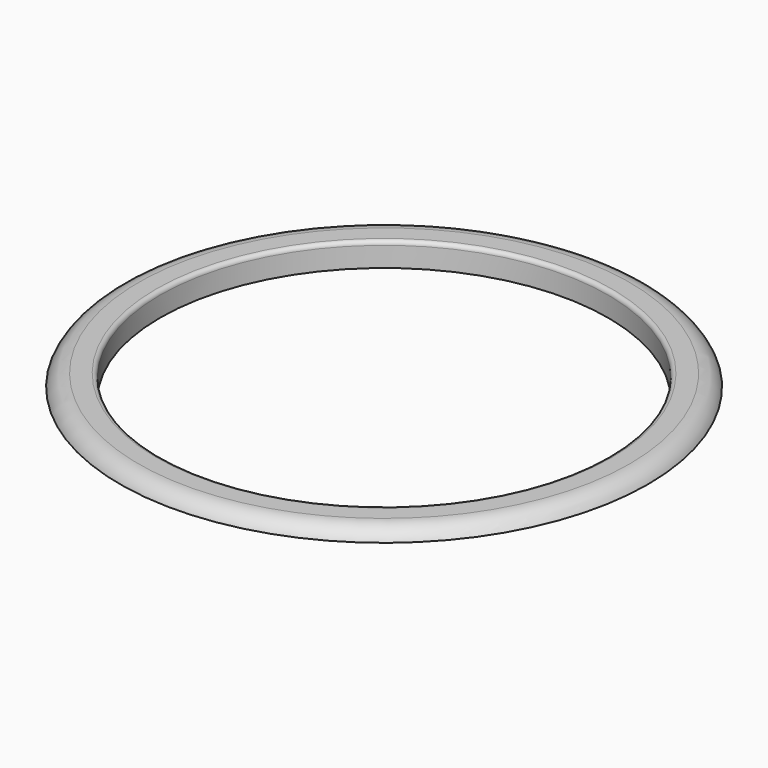
from build123d import *

# Parameters (mm, degrees)
F0_R     = 58
F0_R_2   = 56
F1_DEPTH = 3
F2_R     = 66
F2_R_2   = 58
F2_R_3   = 56
F3_DEPTH = 3
F5_R     = 1


# Not quite as in the source:
# - a fillet or chamfer that OpenCascade refuses, or shapes differently, is made with other operations: its cross-section is extruded or revolved along the edge and cut away or added


with BuildPart() as f1:
    # F0 (on Top) → F1 (new body)
    with BuildSketch(Plane.XY):
        Circle(F0_R)
        Circle(F0_R_2, mode=Mode.SUBTRACT)
    extrude(amount=F1_DEPTH)

    # F2 (on face) → F3 (join)
    with BuildSketch(Plane.XY.offset(3)):
        Circle(F2_R)
        Circle(F2_R_2, mode=Mode.SUBTRACT)
        Circle(F2_R_2)
        Circle(F2_R_3, mode=Mode.SUBTRACT)
    extrude(amount=F3_DEPTH)

    # F4: fillet of radius 5 on 1 edges, made by hand

    # F4_s1 → F4_t2 (revolve, cut)
    with BuildSketch(Plane.XZ):
        with BuildLine():
            ThreePointArc((66, 3), (64.1560370926, 5.1833001327), (61.417424305, 6))
            Line((61.417424305, 6), (66, 6))
            Line((66, 6), (66, 3))
        make_face()
    revolve(axis=Axis((0, 0, 6), (0, 0, 1)), mode=Mode.SUBTRACT)

    # F5
    f5_edges = [f1.edges().sort_by_distance(p)[0] for p in [
        (-56, 0, 6),
    ]]
    fillet(f5_edges, radius=F5_R)


solid = f1.part
